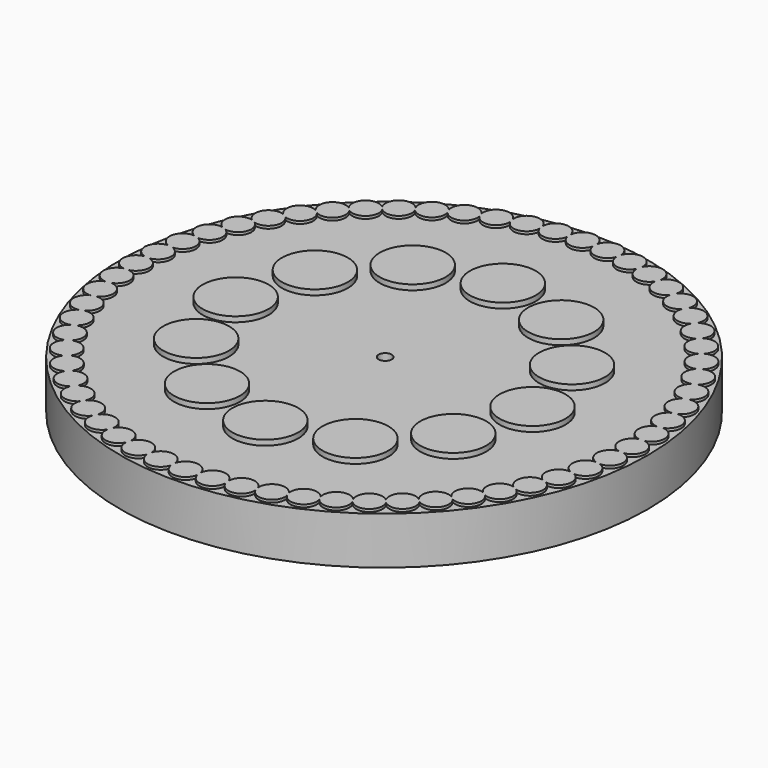
from build123d import *

# Parameters (mm, degrees)
F0_R     = 100
F1_DEPTH = 20
F2_R     = 100
F2_R_2   = 12.5
F3_DEPTH = 1
F4_R     = 100
F4_R_2   = 12.5
F5_DEPTH = 1
F6_R     = 2.5
F7_DEPTH = 25


with BuildPart() as f1:
    # F0 (on Top) → F1 (new body)
    with BuildSketch(Plane.XY):
        Circle(F0_R)
    extrude(amount=-F1_DEPTH)

    # F2 (on face) → F3 (cut)
    with BuildSketch(Plane.XY):
        Circle(F2_R)
        with Locations((-28.1208567321, -48.7067526124)):
            Circle(F2_R_2, mode=Mode.SUBTRACT)
        with Locations((-48.7067526124, -28.1208567321)):
            Circle(F2_R_2, mode=Mode.SUBTRACT)
        with Locations((0, -56.2417134643)):
            Circle(F2_R_2, mode=Mode.SUBTRACT)
        with Locations((28.1208567321, -48.7067526124)):
            Circle(F2_R_2, mode=Mode.SUBTRACT)
        with Locations((48.7067526124, -28.1208567321)):
            Circle(F2_R_2, mode=Mode.SUBTRACT)
        with Locations((-56.2417134643, 0)):
            Circle(F2_R_2, mode=Mode.SUBTRACT)
        with Locations((-48.7067526124, 28.1208567321)):
            Circle(F2_R_2, mode=Mode.SUBTRACT)
        with Locations((-28.1208567321, 48.7067526124)):
            Circle(F2_R_2, mode=Mode.SUBTRACT)
        with Locations((48.7067526124, 28.1208567321)):
            Circle(F2_R_2, mode=Mode.SUBTRACT)
        with Locations((28.1208567321, 48.7067526124)):
            Circle(F2_R_2, mode=Mode.SUBTRACT)
        with Locations((56.2417134643, 0)):
            Circle(F2_R_2, mode=Mode.SUBTRACT)
        with Locations((0, 56.2417134643)):
            Circle(F2_R_2, mode=Mode.SUBTRACT)
    extrude(amount=-F3_DEPTH, mode=Mode.SUBTRACT)

    # F4 (on face) → F5 (cut)
    with BuildSketch(Plane.XY.offset(-1)):
        Circle(F4_R)
        with BuildLine():
            ThreePointArc((-4.9595821255, 94.6344644514), (0, 99), (4.9595821255, 94.6344644514))
            ThreePointArc((4.9595821255, 94.6344644514), (10.3483178635, 98.4576676415), (14.824408157, 93.5976294553))
            ThreePointArc((14.824408157, 93.5976294553), (20.3814178935, 96.8751976426), (24.5436989369, 91.945874469))
            ThreePointArc((24.5436989369, 91.945874469), (24.5394761371, 91.7404233409), (24.5268148705, 91.5353192444))
            ThreePointArc((24.5268148705, 91.5353192444), (30.1421492051, 94.2780374166), (34.0475974712, 89.3993125317))
            ThreePointArc((34.0475974712, 89.3993125317), (34.0257756512, 88.9326841903), (33.9605006676, 88.4701289208))
            ThreePointArc((33.9605006676, 88.4701289208), (39.5816288699, 90.6880273687), (43.2332444491, 85.8732730184))
            ThreePointArc((43.2332444491, 85.8732730184), (43.1801787684, 85.1467464595), (43.0221081128, 84.4356413512))
            ThreePointArc((43.0221081128, 84.4356413512), (48.5985212798, 86.1439748645), (52, 81.4063879557))
            ThreePointArc((52, 81.4063879557), (51.9021312555, 80.4219545382), (51.6123563386, 79.4760592257))
            ThreePointArc((51.6123563386, 79.4760592257), (57.0960904186, 80.695031542), (60.2518137155, 76.0475974712))
            ThreePointArc((60.2518137155, 76.0475974712), (60.0957055062, 74.8079554586), (59.6371287877, 73.6457207638))
            ThreePointArc((59.6371287877, 73.6457207638), (64.9832540899, 74.400156534), (67.8982769977, 69.8556135949))
            ThreePointArc((67.8982769977, 69.8556135949), (67.670652553, 68.3641607597), (67.0085043739, 67.0085043739))
            ThreePointArc((67.0085043739, 67.0085043739), (72.1755762988, 67.3274725288), (74.8556135949, 62.8982769977))
            ThreePointArc((74.8556135949, 62.8982769977), (74.543392165, 61.1591013086), (73.6457207638, 59.6371287877))
            ThreePointArc((73.6457207638, 59.6371287877), (78.5961869304, 59.5535217215), (81.0475974712, 55.2518137155))
            ThreePointArc((81.0475974712, 55.2518137155), (80.637930181, 53.2696821321), (79.4760592257, 51.6123563386))
            ThreePointArc((79.4760592257, 51.6123563386), (84.1766186636, 51.1624297982), (86.4063879557, 47))
            ThreePointArc((86.4063879557, 47), (85.8866930222, 44.7803454072), (84.4356413512, 43.0221081128))
            ThreePointArc((84.4356413512, 43.0221081128), (88.8575519651, 42.2449871089), (90.8732730184, 38.2332444491))
            ThreePointArc((90.8732730184, 38.2332444491), (90.2312702368, 35.7821507659), (88.4701289208, 33.9605006676))
            ThreePointArc((88.4701289208, 33.9605006676), (92.5894600162, 32.8976570847), (94.3993125317, 29.0475974712))
            ThreePointArc((94.3993125317, 29.0475974712), (93.6230569347, 26.371782975), (91.5353192444, 24.5268148705))
            ThreePointArc((91.5353192444, 24.5268148705), (95.3331465186, 23.2215227583), (96.945874469, 19.5436989369))
            ThreePointArc((96.945874469, 19.5436989369), (96.0237890666, 16.6504978491), (93.5976294553, 14.824408157))
            ThreePointArc((93.5976294553, 14.824408157), (97.0601705023, 13.3211829171), (98.4850581646, 9.8256755472))
            ThreePointArc((98.4850581646, 9.8256755472), (97.4059656765, 6.723017931), (94.6344644514, 4.9595821255))
            ThreePointArc((94.6344644514, 4.9595821255), (97.7531534912, 3.3036099757), (99, 0))
            ThreePointArc((99, 0), (97.7531534912, -3.3036099757), (94.6344644514, -4.9595821255))
            ThreePointArc((94.6344644514, -4.9595821255), (97.4059656765, -6.723017931), (98.4850581646, -9.8256755472))
            ThreePointArc((98.4850581646, -9.8256755472), (97.0601705023, -13.3211829171), (93.5976294553, -14.824408157))
            ThreePointArc((93.5976294553, -14.824408157), (96.0237890666, -16.6504978491), (96.945874469, -19.5436989369))
            ThreePointArc((96.945874469, -19.5436989369), (95.3331465186, -23.2215227583), (91.5353192444, -24.5268148705))
            ThreePointArc((91.5353192444, -24.5268148705), (93.6230569347, -26.371782975), (94.3993125317, -29.0475974712))
            ThreePointArc((94.3993125317, -29.0475974712), (92.5894600162, -32.8976570847), (88.4701289208, -33.9605006676))
            ThreePointArc((88.4701289208, -33.9605006676), (90.2312702368, -35.7821507659), (90.8732730184, -38.2332444491))
            ThreePointArc((90.8732730184, -38.2332444491), (88.8575519651, -42.2449871089), (84.4356413512, -43.0221081128))
            ThreePointArc((84.4356413512, -43.0221081128), (85.8866930222, -44.7803454072), (86.4063879557, -47))
            ThreePointArc((86.4063879557, -47), (84.1766186636, -51.1624297982), (79.4760592257, -51.6123563386))
            ThreePointArc((79.4760592257, -51.6123563386), (80.637930181, -53.2696821321), (81.0475974712, -55.2518137155))
            ThreePointArc((81.0475974712, -55.2518137155), (78.5961869304, -59.5535217215), (73.6457207638, -59.6371287877))
            ThreePointArc((73.6457207638, -59.6371287877), (74.543392165, -61.1591013086), (74.8556135949, -62.8982769977))
            ThreePointArc((74.8556135949, -62.8982769977), (72.1755762988, -67.3274725288), (67.0085043739, -67.0085043739))
            ThreePointArc((67.0085043739, -67.0085043739), (67.670652553, -68.3641607597), (67.8982769977, -69.8556135949))
            ThreePointArc((67.8982769977, -69.8556135949), (64.9832540899, -74.400156534), (59.6371287877, -73.6457207638))
            ThreePointArc((59.6371287877, -73.6457207638), (60.0957055062, -74.8079554586), (60.2518137155, -76.0475974712))
            ThreePointArc((60.2518137155, -76.0475974712), (57.0960904186, -80.695031542), (51.6123563386, -79.4760592257))
            ThreePointArc((51.6123563386, -79.4760592257), (51.9021312555, -80.4219545382), (52, -81.4063879557))
            ThreePointArc((52, -81.4063879557), (48.5985212798, -86.1439748645), (43.0221081128, -84.4356413512))
            ThreePointArc((43.0221081128, -84.4356413512), (43.1801787684, -85.1467464595), (43.2332444491, -85.8732730184))
            ThreePointArc((43.2332444491, -85.8732730184), (39.5816288699, -90.6880273687), (33.9605006676, -88.4701289208))
            ThreePointArc((33.9605006676, -88.4701289208), (34.0257756512, -88.9326841903), (34.0475974712, -89.3993125317))
            ThreePointArc((34.0475974712, -89.3993125317), (30.1421492051, -94.2780374166), (24.5268148705, -91.5353192444))
            ThreePointArc((24.5268148705, -91.5353192444), (24.5394761371, -91.7404233409), (24.5436989369, -91.945874469))
            ThreePointArc((24.5436989369, -91.945874469), (20.3814178935, -96.8751976426), (14.824408157, -93.5976294553))
            ThreePointArc((14.824408157, -93.5976294553), (10.3483178635, -98.4576676415), (4.9595821255, -94.6344644514))
            ThreePointArc((4.9595821255, -94.6344644514), (0, -99), (-4.9595821255, -94.6344644514))
            ThreePointArc((-4.9595821255, -94.6344644514), (-10.3483178635, -98.4576676415), (-14.824408157, -93.5976294553))
            ThreePointArc((-14.824408157, -93.5976294553), (-20.583257391, -96.8366124726), (-24.5268148705, -91.5353192444))
            ThreePointArc((-24.5268148705, -91.5353192444), (-30.5926824431, -94.1545951132), (-33.9605006676, -88.4701289208))
            ThreePointArc((-33.9605006676, -88.4701289208), (-40.2669276645, -90.4410003066), (-43.0221081128, -84.4356413512))
            ThreePointArc((-43.0221081128, -84.4356413512), (-49.5, -85.7365149747), (-51.6123563386, -79.4760592257))
            ThreePointArc((-51.6123563386, -79.4760592257), (-58.190739977, -80.0926824431), (-59.6371287877, -73.6457207638))
            ThreePointArc((-59.6371287877, -73.6457207638), (-66.2439300295, -73.5713377223), (-67.0085043739, -67.0085043739))
            ThreePointArc((-67.0085043739, -67.0085043739), (-73.5713377223, -66.2439300295), (-73.6457207638, -59.6371287877))
            ThreePointArc((-73.6457207638, -59.6371287877), (-80.0926824431, -58.190739977), (-79.4760592257, -51.6123563386))
            ThreePointArc((-79.4760592257, -51.6123563386), (-85.7365149747, -49.5), (-84.4356413512, -43.0221081128))
            ThreePointArc((-84.4356413512, -43.0221081128), (-90.4410003066, -40.2669276645), (-88.4701289208, -33.9605006676))
            ThreePointArc((-88.4701289208, -33.9605006676), (-94.1545951132, -30.5926824431), (-91.5353192444, -24.5268148705))
            ThreePointArc((-91.5353192444, -24.5268148705), (-96.8366124726, -20.583257391), (-93.5976294553, -14.824408157))
            ThreePointArc((-93.5976294553, -14.824408157), (-98.4576676415, -10.3483178635), (-94.6344644514, -4.9595821255))
            ThreePointArc((-94.6344644514, -4.9595821255), (-99, 0), (-94.6344644514, 4.9595821255))
            ThreePointArc((-94.6344644514, 4.9595821255), (-98.4576676415, 10.3483178635), (-93.5976294553, 14.824408157))
            ThreePointArc((-93.5976294553, 14.824408157), (-96.8366124726, 20.583257391), (-91.5353192444, 24.5268148705))
            ThreePointArc((-91.5353192444, 24.5268148705), (-94.1545951132, 30.5926824431), (-88.4701289208, 33.9605006676))
            ThreePointArc((-88.4701289208, 33.9605006676), (-90.4410003066, 40.2669276645), (-84.4356413512, 43.0221081128))
            ThreePointArc((-84.4356413512, 43.0221081128), (-85.7365149747, 49.5), (-79.4760592257, 51.6123563386))
            ThreePointArc((-79.4760592257, 51.6123563386), (-80.0926824431, 58.190739977), (-73.6457207638, 59.6371287877))
            ThreePointArc((-73.6457207638, 59.6371287877), (-73.5713377223, 66.2439300295), (-67.0085043739, 67.0085043739))
            ThreePointArc((-67.0085043739, 67.0085043739), (-66.2439300295, 73.5713377223), (-59.6371287877, 73.6457207638))
            ThreePointArc((-59.6371287877, 73.6457207638), (-58.190739977, 80.0926824431), (-51.6123563386, 79.4760592257))
            ThreePointArc((-51.6123563386, 79.4760592257), (-49.5, 85.7365149747), (-43.0221081128, 84.4356413512))
            ThreePointArc((-43.0221081128, 84.4356413512), (-40.2669276645, 90.4410003066), (-33.9605006676, 88.4701289208))
            ThreePointArc((-33.9605006676, 88.4701289208), (-30.5926824431, 94.1545951132), (-24.5268148705, 91.5353192444))
            ThreePointArc((-24.5268148705, 91.5353192444), (-20.583257391, 96.8366124726), (-14.824408157, 93.5976294553))
            ThreePointArc((-14.824408157, 93.5976294553), (-10.3483178635, 98.4576676415), (-4.9595821255, 94.6344644514))
        make_face(mode=Mode.SUBTRACT)
        with BuildLine():
            ThreePointArc((14.544966327, 91.8333031783), (9.3030332308, 88.5124486878), (4.8660934216, 92.8505937132))
            ThreePointArc((4.8660934216, 92.8505937132), (0, 89), (-4.8660934216, 92.8505937132))
            ThreePointArc((-4.8660934216, 92.8505937132), (-9.3030332308, 88.5124486878), (-14.544966327, 91.8333031783))
            ThreePointArc((-14.544966327, 91.8333031783), (-18.5041404828, 87.0551364653), (-24.0644815377, 89.8098677564))
            ThreePointArc((-24.0644815377, 89.8098677564), (-24.0518202711, 89.6047636598), (-24.0475974712, 89.3993125317))
            ThreePointArc((-24.0475974712, 89.3993125317), (-27.6992130504, 84.5845581814), (-33.3203412527, 86.8024566294))
            ThreePointArc((-33.3203412527, 86.8024566294), (-33.2550662692, 86.3399013598), (-33.2332444491, 85.8732730184))
            ThreePointArc((-33.2332444491, 85.8732730184), (-36.6347231693, 81.1356861097), (-42.2111363363, 82.8440196229))
            ThreePointArc((-42.2111363363, 82.8440196229), (-42.0530656807, 82.1329145146), (-42, 81.4063879557))
            ThreePointArc((-42, 81.4063879557), (-45.1557232969, 76.7589538849), (-50.6394573769, 77.9779262013))
            ThreePointArc((-50.6394573769, 77.9779262013), (-50.34968246, 77.0320308888), (-50.2518137155, 76.0475974712))
            ThreePointArc((-50.2518137155, 76.0475974712), (-53.1668366233, 71.5030545322), (-58.5129619256, 72.2574903023))
            ThreePointArc((-58.5129619256, 72.2574903023), (-58.054385207, 71.0952556075), (-57.8982769977, 69.8556135949))
            ThreePointArc((-57.8982769977, 69.8556135949), (-60.5783142938, 65.4264180638), (-65.7453862187, 65.7453862187))
            ThreePointArc((-65.7453862187, 65.7453862187), (-65.0832380396, 64.3897298329), (-64.8556135949, 62.8982769977))
            ThreePointArc((-64.8556135949, 62.8982769977), (-67.3070241357, 58.5965689918), (-72.2574903023, 58.5129619256))
            ThreePointArc((-72.2574903023, 58.5129619256), (-71.3598189011, 56.9909894046), (-71.0475974712, 55.2518137155))
            ThreePointArc((-71.0475974712, 55.2518137155), (-73.2773667634, 51.0893839173), (-77.9779262013, 50.6394573769))
            ThreePointArc((-77.9779262013, 50.6394573769), (-76.816055246, 48.9821315834), (-76.4063879557, 47))
            ThreePointArc((-76.4063879557, 47), (-78.422109009, 42.9882573403), (-82.8440196229, 42.2111363363))
            ThreePointArc((-82.8440196229, 42.2111363363), (-81.3929679519, 40.4528990419), (-80.8732730184, 38.2332444491))
            ThreePointArc((-80.8732730184, 38.2332444491), (-82.6831255339, 34.3831848356), (-86.8024566294, 33.3203412527))
            ThreePointArc((-86.8024566294, 33.3203412527), (-85.0413153133, 31.4986911545), (-84.3993125317, 29.0475974712))
            ThreePointArc((-84.3993125317, 29.0475974712), (-86.0120404821, 25.3697736498), (-89.8098677564, 24.0644815377))
            ThreePointArc((-89.8098677564, 24.0644815377), (-87.722130066, 22.2195134331), (-86.945874469, 19.5436989369))
            ThreePointArc((-86.945874469, 19.5436989369), (-88.3707621313, 16.0481915669), (-91.8333031783, 14.544966327))
            ThreePointArc((-91.8333031783, 14.544966327), (-89.407143567, 12.7188766349), (-88.4850581646, 9.8256755472))
            ThreePointArc((-88.4850581646, 9.8256755472), (-89.7319046734, 6.5220655715), (-92.8505937132, 4.8660934216))
            ThreePointArc((-92.8505937132, 4.8660934216), (-90.0790924881, 3.1026576162), (-89, 0))
            ThreePointArc((-89, 0), (-90.0790924881, -3.1026576162), (-92.8505937132, -4.8660934216))
            ThreePointArc((-92.8505937132, -4.8660934216), (-89.7319046734, -6.5220655715), (-88.4850581646, -9.8256755472))
            ThreePointArc((-88.4850581646, -9.8256755472), (-89.407143567, -12.7188766349), (-91.8333031783, -14.544966327))
            ThreePointArc((-91.8333031783, -14.544966327), (-88.3707621313, -16.0481915669), (-86.945874469, -19.5436989369))
            ThreePointArc((-86.945874469, -19.5436989369), (-87.722130066, -22.2195134331), (-89.8098677564, -24.0644815377))
            ThreePointArc((-89.8098677564, -24.0644815377), (-86.0120404821, -25.3697736498), (-84.3993125317, -29.0475974712))
            ThreePointArc((-84.3993125317, -29.0475974712), (-85.0413153133, -31.4986911545), (-86.8024566294, -33.3203412527))
            ThreePointArc((-86.8024566294, -33.3203412527), (-82.6831255339, -34.3831848356), (-80.8732730184, -38.2332444491))
            ThreePointArc((-80.8732730184, -38.2332444491), (-81.3929679519, -40.4528990419), (-82.8440196229, -42.2111363363))
            ThreePointArc((-82.8440196229, -42.2111363363), (-78.422109009, -42.9882573403), (-76.4063879557, -47))
            ThreePointArc((-76.4063879557, -47), (-76.816055246, -48.9821315834), (-77.9779262013, -50.6394573769))
            ThreePointArc((-77.9779262013, -50.6394573769), (-73.2773667634, -51.0893839173), (-71.0475974712, -55.2518137155))
            ThreePointArc((-71.0475974712, -55.2518137155), (-71.3598189011, -56.9909894046), (-72.2574903023, -58.5129619256))
            ThreePointArc((-72.2574903023, -58.5129619256), (-67.3070241357, -58.5965689918), (-64.8556135949, -62.8982769977))
            ThreePointArc((-64.8556135949, -62.8982769977), (-65.0832380396, -64.3897298329), (-65.7453862187, -65.7453862187))
            ThreePointArc((-65.7453862187, -65.7453862187), (-60.5783142938, -65.4264180638), (-57.8982769977, -69.8556135949))
            ThreePointArc((-57.8982769977, -69.8556135949), (-58.054385207, -71.0952556075), (-58.5129619256, -72.2574903023))
            ThreePointArc((-58.5129619256, -72.2574903023), (-53.1668366233, -71.5030545322), (-50.2518137155, -76.0475974712))
            ThreePointArc((-50.2518137155, -76.0475974712), (-50.34968246, -77.0320308888), (-50.6394573769, -77.9779262013))
            ThreePointArc((-50.6394573769, -77.9779262013), (-45.1557232969, -76.7589538849), (-42, -81.4063879557))
            ThreePointArc((-42, -81.4063879557), (-42.0530656807, -82.1329145146), (-42.2111363363, -82.8440196229))
            ThreePointArc((-42.2111363363, -82.8440196229), (-36.6347231693, -81.1356861097), (-33.2332444491, -85.8732730184))
            ThreePointArc((-33.2332444491, -85.8732730184), (-33.2550662692, -86.3399013598), (-33.3203412527, -86.8024566294))
            ThreePointArc((-33.3203412527, -86.8024566294), (-27.6992130504, -84.5845581814), (-24.0475974712, -89.3993125317))
            ThreePointArc((-24.0475974712, -89.3993125317), (-24.0518202711, -89.6047636598), (-24.0644815377, -89.8098677564))
            ThreePointArc((-24.0644815377, -89.8098677564), (-18.5041404828, -87.0551364653), (-14.544966327, -91.8333031783))
            ThreePointArc((-14.544966327, -91.8333031783), (-9.3030332308, -88.5124486878), (-4.8660934216, -92.8505937132))
            ThreePointArc((-4.8660934216, -92.8505937132), (0, -89), (4.8660934216, -92.8505937132))
            ThreePointArc((4.8660934216, -92.8505937132), (9.3030332308, -88.5124486878), (14.544966327, -91.8333031783))
            ThreePointArc((14.544966327, -91.8333031783), (18.5041404828, -87.0551364653), (24.0644815377, -89.8098677564))
            ThreePointArc((24.0644815377, -89.8098677564), (27.5025124994, -84.6440299503), (33.3203412527, -86.8024566294))
            ThreePointArc((33.3203412527, -86.8024566294), (36.1995612337, -81.3055457302), (42.2111363363, -82.8440196229))
            ThreePointArc((42.2111363363, -82.8440196229), (44.5, -77.0762609368), (50.6394573769, -77.9779262013))
            ThreePointArc((50.6394573769, -77.9779262013), (52.312887454, -72.0025124994), (58.5129619256, -72.2574903023))
            ThreePointArc((58.5129619256, -72.2574903023), (59.5526239659, -66.1398894675), (65.7453862187, -65.7453862187))
            ThreePointArc((65.7453862187, -65.7453862187), (66.1398894675, -59.5526239659), (72.2574903023, -58.5129619256))
            ThreePointArc((72.2574903023, -58.5129619256), (72.0025124994, -52.312887454), (77.9779262013, -50.6394573769))
            ThreePointArc((77.9779262013, -50.6394573769), (77.0762609368, -44.5), (82.8440196229, -42.2111363363))
            ThreePointArc((82.8440196229, -42.2111363363), (81.3055457302, -36.1995612337), (86.8024566294, -33.3203412527))
            ThreePointArc((86.8024566294, -33.3203412527), (84.6440299503, -27.5025124994), (89.8098677564, -24.0644815377))
            ThreePointArc((89.8098677564, -24.0644815377), (87.0551364653, -18.5041404828), (91.8333031783, -14.544966327))
            ThreePointArc((91.8333031783, -14.544966327), (88.5124486878, -9.3030332308), (92.8505937132, -4.8660934216))
            ThreePointArc((92.8505937132, -4.8660934216), (89, 0), (92.8505937132, 4.8660934216))
            ThreePointArc((92.8505937132, 4.8660934216), (88.5124486878, 9.3030332308), (91.8333031783, 14.544966327))
            ThreePointArc((91.8333031783, 14.544966327), (87.0551364653, 18.5041404828), (89.8098677564, 24.0644815377))
            ThreePointArc((89.8098677564, 24.0644815377), (84.6440299503, 27.5025124994), (86.8024566294, 33.3203412527))
            ThreePointArc((86.8024566294, 33.3203412527), (81.3055457302, 36.1995612337), (82.8440196229, 42.2111363363))
            ThreePointArc((82.8440196229, 42.2111363363), (77.0762609368, 44.5), (77.9779262013, 50.6394573769))
            ThreePointArc((77.9779262013, 50.6394573769), (72.0025124994, 52.312887454), (72.2574903023, 58.5129619256))
            ThreePointArc((72.2574903023, 58.5129619256), (66.1398894675, 59.5526239659), (65.7453862187, 65.7453862187))
            ThreePointArc((65.7453862187, 65.7453862187), (59.5526239659, 66.1398894675), (58.5129619256, 72.2574903023))
            ThreePointArc((58.5129619256, 72.2574903023), (52.312887454, 72.0025124994), (50.6394573769, 77.9779262013))
            ThreePointArc((50.6394573769, 77.9779262013), (44.5, 77.0762609368), (42.2111363363, 82.8440196229))
            ThreePointArc((42.2111363363, 82.8440196229), (36.1995612337, 81.3055457302), (33.3203412527, 86.8024566294))
            ThreePointArc((33.3203412527, 86.8024566294), (27.5025124994, 84.6440299503), (24.0644815377, 89.8098677564))
            ThreePointArc((24.0644815377, 89.8098677564), (18.5041404828, 87.0551364653), (14.544966327, 91.8333031783))
        make_face()
        with Locations((-28.1208567321, -48.7067526124)):
            Circle(F4_R_2, mode=Mode.SUBTRACT)
        with Locations((-48.7067526124, -28.1208567321)):
            Circle(F4_R_2, mode=Mode.SUBTRACT)
        with Locations((0, -56.2417134643)):
            Circle(F4_R_2, mode=Mode.SUBTRACT)
        with Locations((28.1208567321, -48.7067526124)):
            Circle(F4_R_2, mode=Mode.SUBTRACT)
        with Locations((48.7067526124, -28.1208567321)):
            Circle(F4_R_2, mode=Mode.SUBTRACT)
        with Locations((-56.2417134643, 0)):
            Circle(F4_R_2, mode=Mode.SUBTRACT)
        with Locations((-48.7067526124, 28.1208567321)):
            Circle(F4_R_2, mode=Mode.SUBTRACT)
        with Locations((-28.1208567321, 48.7067526124)):
            Circle(F4_R_2, mode=Mode.SUBTRACT)
        with Locations((48.7067526124, 28.1208567321)):
            Circle(F4_R_2, mode=Mode.SUBTRACT)
        with Locations((28.1208567321, 48.7067526124)):
            Circle(F4_R_2, mode=Mode.SUBTRACT)
        with Locations((56.2417134643, 0)):
            Circle(F4_R_2, mode=Mode.SUBTRACT)
        with Locations((0, 56.2417134643)):
            Circle(F4_R_2, mode=Mode.SUBTRACT)
    extrude(amount=-F5_DEPTH, mode=Mode.SUBTRACT)

    # F6 (on face) → F7 (cut)
    with BuildSketch(Plane.XY.offset(-2)):
        with Locations((0, 0.5334001524)):
            Circle(F6_R)
    extrude(amount=-F7_DEPTH, mode=Mode.SUBTRACT)


solid = f1.part
